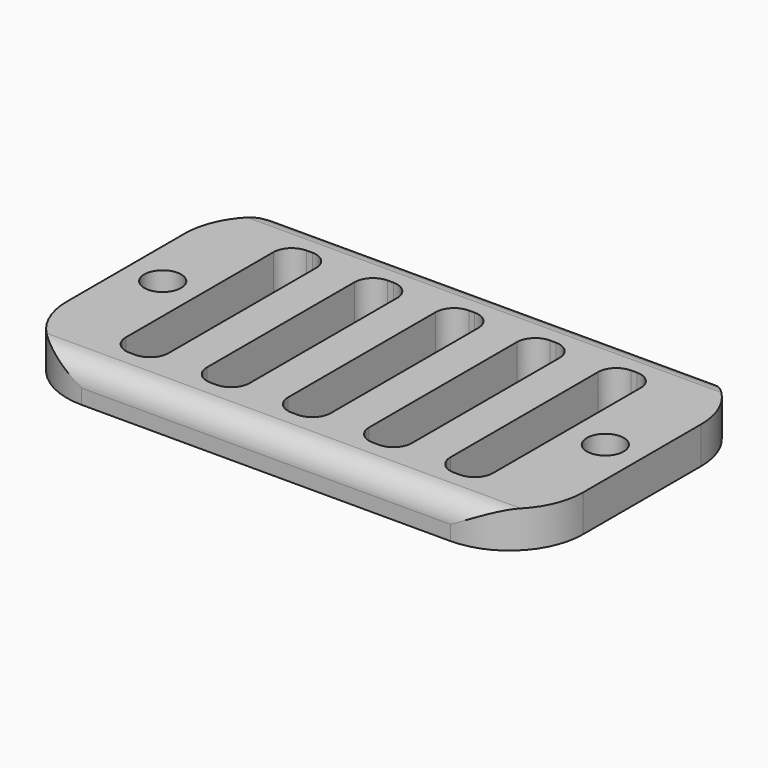
from build123d import *

# Parameters (mm, degrees)
F0_W        = 70
F0_H        = 40
F0_R        = 2.5
F1_DEPTH    = 5
F2_R        = 10
F3_T1_DEPTH = 65


# Not quite as in the source:
# - a fillet or chamfer that OpenCascade refuses, or shapes differently, is made with other operations: its cross-section is extruded or revolved along the edge and cut away or added


with BuildPart() as f1:
    # F0 (on Top) → F1 (new body)
    with BuildSketch(Plane.XY):
        Rectangle(F0_W, F0_H)
        with Locations((-30, 0)):
            Circle(F0_R, mode=Mode.SUBTRACT)
        with BuildLine():
            ThreePointArc((-25, 12.5), (-24.267766953, 14.267766953), (-22.5, 15))
            Line((-22.5, 15), (-21.7131334842, 15))
            ThreePointArc((-21.7131334842, 15), (-19.9453665312, 14.267766953), (-19.2131334842, 12.5))
            Line((-19.2131334842, 12.5), (-19.2131334842, -12.5))
            ThreePointArc((-19.2131334842, -12.5), (-19.9453665312, -14.267766953), (-21.7131334842, -15))
            Line((-21.7131334842, -15), (-22.5, -15))
            ThreePointArc((-22.5, -15), (-24.267766953, -14.267766953), (-25, -12.5))
            Line((-25, -12.5), (-25, 12.5))
        make_face(mode=Mode.SUBTRACT)
        with BuildLine():
            Line((-14, -12.5), (-14, 12.5))
            ThreePointArc((-14, 12.5), (-13.267766953, 14.267766953), (-11.5, 15))
            Line((-11.5, 15), (-10.7131334842, 15))
            ThreePointArc((-10.7131334842, 15), (-8.9453665312, 14.267766953), (-8.2131334842, 12.5))
            Line((-8.2131334842, 12.5), (-8.2131334842, -12.5))
            ThreePointArc((-8.2131334842, -12.5), (-8.9453665312, -14.267766953), (-10.7131334842, -15))
            Line((-10.7131334842, -15), (-11.5, -15))
            ThreePointArc((-11.5, -15), (-13.267766953, -14.267766953), (-14, -12.5))
        make_face(mode=Mode.SUBTRACT)
        with BuildLine():
            Line((-3, -12.5), (-3, 12.5))
            ThreePointArc((-3, 12.5), (-2.267766953, 14.267766953), (-0.5, 15))
            Line((-0.5, 15), (0.2868665158, 15))
            ThreePointArc((0.2868665158, 15), (2.0546334688, 14.267766953), (2.7868665158, 12.5))
            Line((2.7868665158, 12.5), (2.7868665158, -12.5))
            ThreePointArc((2.7868665158, -12.5), (2.0546334688, -14.267766953), (0.2868665158, -15))
            Line((0.2868665158, -15), (-0.5, -15))
            ThreePointArc((-0.5, -15), (-2.267766953, -14.267766953), (-3, -12.5))
        make_face(mode=Mode.SUBTRACT)
        with BuildLine():
            Line((8, -12.5), (8, 12.5))
            ThreePointArc((8, 12.5), (8.732233047, 14.267766953), (10.5, 15))
            Line((10.5, 15), (11.2868665158, 15))
            ThreePointArc((11.2868665158, 15), (13.0546334688, 14.267766953), (13.7868665158, 12.5))
            Line((13.7868665158, 12.5), (13.7868665158, -12.5))
            ThreePointArc((13.7868665158, -12.5), (13.0546334688, -14.267766953), (11.2868665158, -15))
            Line((11.2868665158, -15), (10.5, -15))
            ThreePointArc((10.5, -15), (8.732233047, -14.267766953), (8, -12.5))
        make_face(mode=Mode.SUBTRACT)
        with BuildLine():
            Line((19, -12.5), (19, 12.5))
            ThreePointArc((19, 12.5), (19.732233047, 14.267766953), (21.5, 15))
            Line((21.5, 15), (22.2868665158, 15))
            ThreePointArc((22.2868665158, 15), (24.0546334688, 14.267766953), (24.7868665158, 12.5))
            Line((24.7868665158, 12.5), (24.7868665158, -12.5))
            ThreePointArc((24.7868665158, -12.5), (24.0546334688, -14.267766953), (22.2868665158, -15))
            Line((22.2868665158, -15), (21.5, -15))
            ThreePointArc((21.5, -15), (19.732233047, -14.267766953), (19, -12.5))
        make_face(mode=Mode.SUBTRACT)
        with Locations((30, 0)):
            Circle(F0_R, mode=Mode.SUBTRACT)
    extrude(amount=F1_DEPTH)

    # F2
    f2_edges = [f1.edges().sort_by_distance(p)[0] for p in [
        (-35, 20, 2.5),
        (-35, -20, 2.5),
        (35, -20, 2.5),
        (35, 20, 2.5),
    ]]
    fillet(f2_edges, radius=F2_R)

    # F3: fillet of radius 3 on 2 edges, made by hand

    # F3_s2 → F3_t1 (cut)
    with BuildSketch(Plane.YZ.offset(-32.5)):
        with BuildLine():
            ThreePointArc((-17, 5), (-19.1213203436, 4.1213203436), (-20, 2))
            Line((-20, 2), (-20, 5))
            Line((-20, 5), (-17, 5))
        make_face()
        with BuildLine():
            ThreePointArc((20, 2), (19.1213203436, 4.1213203436), (17, 5))
            Line((17, 5), (20, 5))
            Line((20, 5), (20, 2))
        make_face()
    extrude(amount=F3_T1_DEPTH, mode=Mode.SUBTRACT)


solid = f1.part
